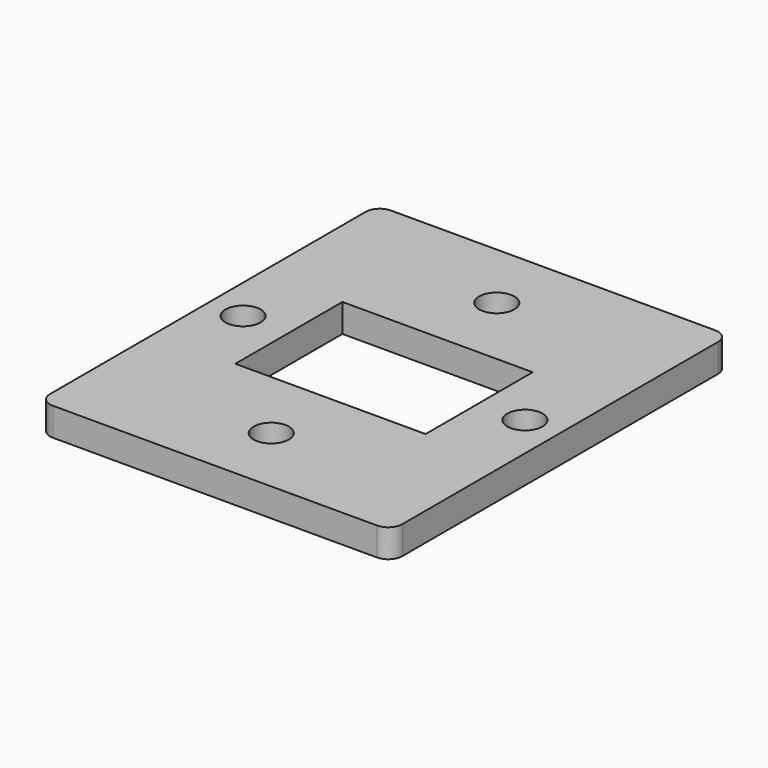
from build123d import *

# Parameters (mm, degrees)
F0_W     = 50
F0_H     = 60
F0_R     = 2.5
F0_W_2   = 27
F0_H_2   = 19
F1_DEPTH = 4
F2_R     = 2


with BuildPart() as f1:
    # F0 (on Top) → F1 (new body)
    with BuildSketch(Plane.XY):
        Rectangle(F0_W, F0_H)
        with Locations((0, -20)):
            Circle(F0_R, mode=Mode.SUBTRACT)
        with Locations((-20, 0)):
            Circle(F0_R, mode=Mode.SUBTRACT)
        Rectangle(F0_W_2, F0_H_2, mode=Mode.SUBTRACT)
        with Locations((20, 0)):
            Circle(F0_R, mode=Mode.SUBTRACT)
        with Locations((0, 20)):
            Circle(F0_R, mode=Mode.SUBTRACT)
    extrude(amount=F1_DEPTH)

    # F2
    f2_edges = [f1.edges().sort_by_distance(p)[0] for p in [
        (25, 30, 2),
        (25, -30, 2),
        (-25, 30, 2),
        (-25, -30, 2),
    ]]
    fillet(f2_edges, radius=F2_R)


solid = f1.part
